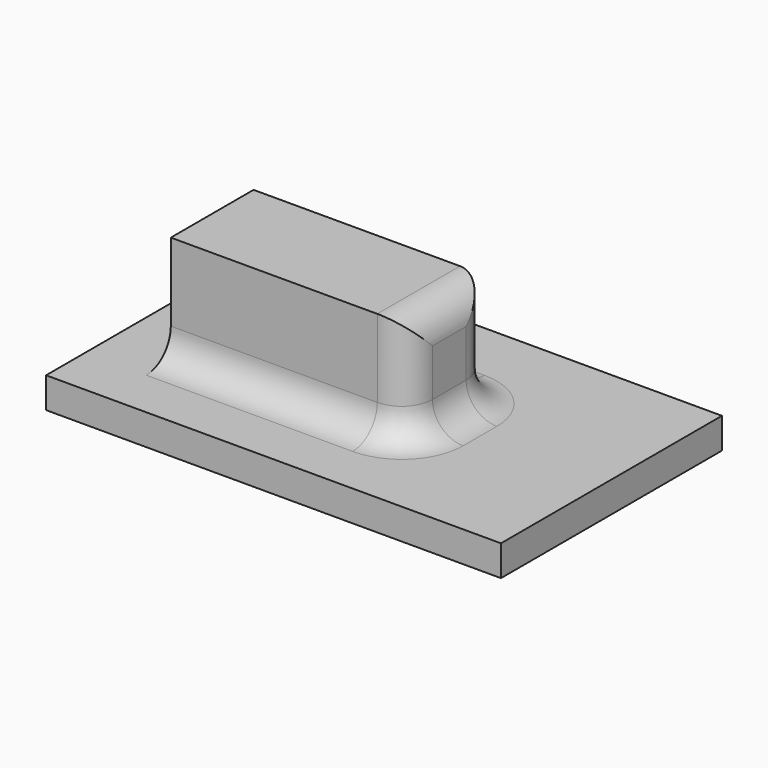
from build123d import *

# Parameters (mm, degrees)
F0_W     = 74.1118490696
F0_H     = 45.0000055134
F1_DEPTH = 5
F3_W     = 38.6348655447
F3_H     = 16.8519383296
F4_DEPTH = 17.7
F5_R     = 5


with BuildPart() as f1:
    # F0 (on Top) → F1 (new body)
    with BuildSketch(Plane.XY):
        with Locations((37.0559245348, 22.5000027567)):
            Rectangle(F0_W, F0_H)
    extrude(amount=F1_DEPTH)

    # F3 (on face) → F4 (join)
    with BuildSketch(Plane.XY.offset(5)):
        with Locations((29.2525482364, 21.4091469534)):
            Rectangle(F3_W, F3_H)
    extrude(amount=F4_DEPTH)

    # F5
    f5_edges = [f1.edges().sort_by_distance(p)[0] for p in [
        (48.569981, 12.983178, 13.85),
        (48.569981, 29.835116, 13.85),
        (48.569981, 21.409147, 5),
        (48.569981, 21.409147, 22.7),
        (29.252548, 12.983178, 5),
        (29.252548, 29.835116, 5),
    ]]
    fillet(f5_edges, radius=F5_R)


solid = f1.part
